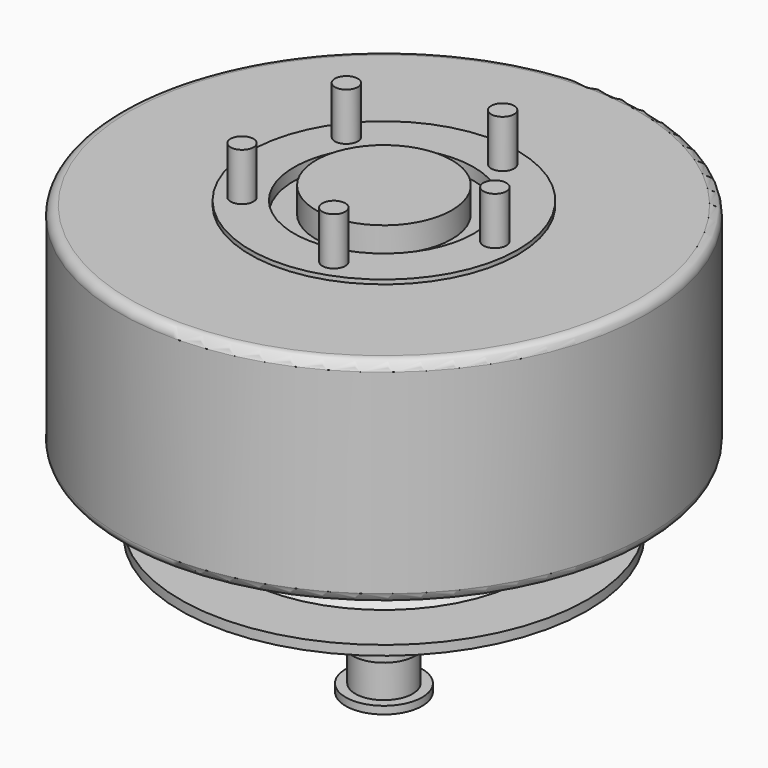
from build123d import *

# Parameters (mm, degrees)
F0_R      = 138
F1_DEPTH  = 112
F2_R      = 70
F3_DEPTH  = 2.25
F4_R      = 5
F5_R      = 47
F6_DEPTH  = 6.3
F8_R      = 6
F9_DEPTH  = 25
F7_R      = 35.5
F10_DEPTH = 13.3
F11_R     = 47.5
F12_DEPTH = 15
F13_R     = 26.4
F14_DEPTH = 6
F15_R     = 3.5
F16_DEPTH = 12
F17_R     = 16.5
F18_DEPTH = 69
F19_R     = 15
F20_DEPTH = 22
F21_R     = 10.5
F22_DEPTH = 251.251
F26_DEPTH = 2.6
F27_R     = 20
F27_R_2   = 15
F28_DEPTH = 4
F31_R     = 3.5
F32_DEPTH = 25


with BuildPart() as f1:
    # F0 (on Top) → F1 (new body)
    with BuildSketch(Plane.XY):
        Circle(F0_R)
    extrude(amount=F1_DEPTH)

    # F2 (on face) → F3 (join)
    with BuildSketch(Plane.XY.offset(112)):
        Circle(F2_R)
    extrude(amount=F3_DEPTH)

    # F4
    f4_edges = [f1.edges().sort_by_distance(p)[0] for p in [
        (138, 0, 56),
        (-138, 0, 0),
        (-138, 0, 112),
    ]]
    fillet(f4_edges, radius=F4_R)

    # F5 (on face) → F6 (cut)
    with BuildSketch(Plane.XY.offset(114.25)):
        Circle(F5_R)
    extrude(amount=-F6_DEPTH, mode=Mode.SUBTRACT)

    # F8 (on face) → F9 (join)
    with BuildSketch(Plane.XY.offset(114.25)):
        with Locations((58, 0)):
            Circle(F8_R)
        with Locations((17.9229856737, 55.1612779451)):
            Circle(F8_R)
        with Locations((-46.9229856737, 34.091544633)):
            Circle(F8_R)
        with Locations((-46.9229856737, -34.091544633)):
            Circle(F8_R)
        with Locations((17.9229856737, -55.1612779451)):
            Circle(F8_R)
    extrude(amount=F9_DEPTH)

    # F7 (on face) → F10 (join)
    with BuildSketch(Plane.XY.offset(107.95)):
        Circle(F7_R)
    extrude(amount=F10_DEPTH)

    # F11 (on face) → F12 (join)
    with BuildSketch(Plane(origin=(0, 0, 0), x_dir=(1, 0, 0), z_dir=(0, 0, -1))):
        Circle(F11_R)
    extrude(amount=F12_DEPTH)

    # F13 (on face) → F14 (join)
    with BuildSketch(Plane(origin=(0, 0, -15), x_dir=(1, 0, 0), z_dir=(0, 0, -1))):
        Circle(F13_R)
    extrude(amount=F14_DEPTH)

    # F15 (on face) → F16 (cut)
    with BuildSketch(Plane(origin=(0, 0, -15), x_dir=(1, 0, 0), z_dir=(0, 0, -1))):
        with Locations((33.5041616609, 14.4817523593)):
            Circle(F15_R)
        with Locations((-14.4817523593, 33.5041616609)):
            Circle(F15_R)
        with Locations((-33.5041616609, -14.4817523593)):
            Circle(F15_R)
        with Locations((14.4817523593, -33.5041616609)):
            Circle(F15_R)
    extrude(amount=-F16_DEPTH, mode=Mode.SUBTRACT)


with BuildPart() as f18:
    # F17 (on face) → F18 (new body)
    with BuildSketch(Plane(origin=(0, 0, -21), x_dir=(1, 0, 0), z_dir=(0, 0, -1))):
        Circle(F17_R)
    extrude(amount=F18_DEPTH)

    # F19 (on face) → F20 (join)
    with BuildSketch(Plane(origin=(0, 0, -90), x_dir=(1, 0, 0), z_dir=(0, 0, -1))):
        Circle(F19_R)
    extrude(amount=F20_DEPTH)

    # F21 (on face) → F22 (cut, through all)
    with BuildSketch(Plane(origin=(0, 0, -112), x_dir=(1, 0, 0), z_dir=(0, 0, -1))):
        Circle(F21_R)
    extrude(amount=-F22_DEPTH, mode=Mode.SUBTRACT)

    # F25 (on line) → F26 (cut)
    with BuildSketch(Plane(origin=(-16.5, 0, 0), x_dir=(0, -1, 0), z_dir=(-1, 0, 0))):
        with BuildLine():
            ThreePointArc((-4, -60), (0, -64), (4, -60))
            Line((4, -60), (4, -38))
            ThreePointArc((4, -38), (0, -34), (-4, -38))
            Line((-4, -38), (-4, -60))
        make_face()
    extrude(amount=-F26_DEPTH, mode=Mode.SUBTRACT)


with BuildPart() as f28:
    # F27 (on face) → F28 (new body)
    with BuildSketch(Plane(origin=(0, 0, -112), x_dir=(1, 0, 0), z_dir=(0, 0, -1))):
        Circle(F27_R)
        Circle(F27_R_2, mode=Mode.SUBTRACT)
    extrude(amount=-F28_DEPTH)


with BuildPart() as f30:
    # F29 (on Front) → F30 (revolve)
    with BuildSketch(Plane.XZ):
        Polygon((44.4, -15), (26.4, -15), (26.4, -20), (42.3000603914, -20), (73.4, -40), (106.4, -40), (106.4, -35), (75.4999396086, -35), align=None)
    revolve(axis=Axis((0, 0, -37.7042032778), (0, 0, -1)))

    # F31 (on face) → F32 (cut)
    with BuildSketch(Plane(origin=(0, 0, -20), x_dir=(1, 0, 0), z_dir=(0, 0, -1))):
        with Locations((33.5041616609, 14.4817523593)):
            Circle(F31_R)
        with Locations((-14.4817523593, 33.5041616609)):
            Circle(F31_R)
        with Locations((-33.5041616609, -14.4817523593)):
            Circle(F31_R)
        with Locations((14.4817523593, -33.5041616609)):
            Circle(F31_R)
    extrude(amount=-F32_DEPTH, mode=Mode.SUBTRACT)


solid = Compound([f1.part, f18.part, f28.part, f30.part])
